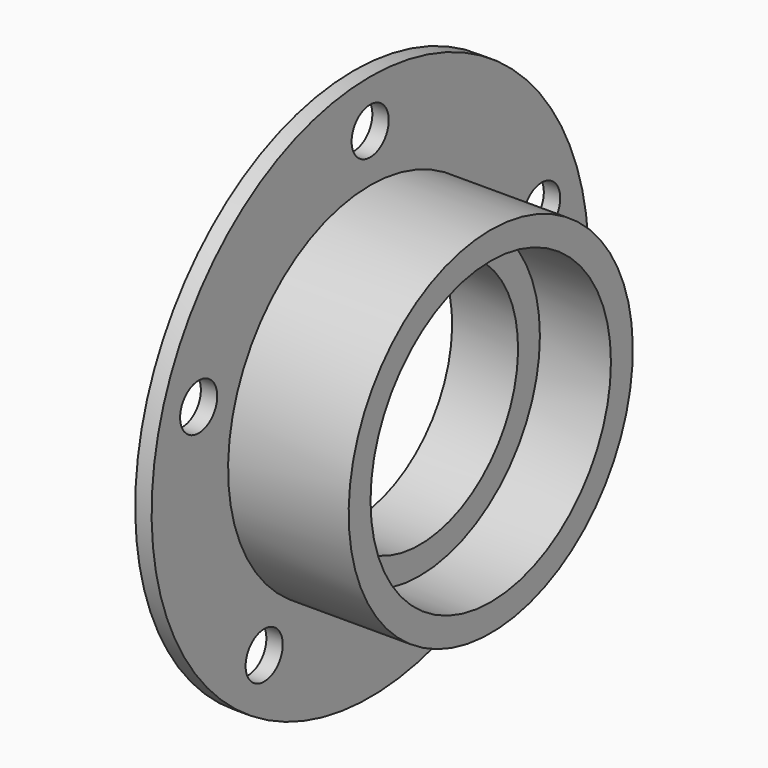
from build123d import *

# Parameters (mm, degrees)
F3_D     = 8.5
F3_DEPTH = 49.5
F3_TIP   = 2.5536576309


# Not quite as in the source:
# - a feature names something its author has since deleted; it is built from what else it names


with BuildPart() as f1:
    # F0 (on Front) → F1 (revolve)
    with BuildSketch(Plane.XZ):
        Polygon((-15.4332816247, 27.5), (-2.4332816247, 27.5), (-2.4332816247, 32.5), (-24.5, 32.5), (-24.5, 50), (-27.5, 50), (-27.5, 22.5), (-15.4332816247, 22.5), align=None)
    revolve(axis=Axis((-62.9697144032, 0, 0), (-1, 0, 0)))

    # F3
    with Locations(Plane(origin=(-27.5, 0, 0), x_dir=(0, -1, 0), z_dir=(-1, 0, 0))):
        with Locations((0, 41.25), (39.2310812972, 12.746951018), (24.2461416571, -33.371951018), (-24.2461416571, -33.371951018), (-39.2310812972, 12.746951018)):
            Hole(F3_D / 2, depth=F3_DEPTH)
            with Locations((0, 0, -(F3_DEPTH + F3_TIP / 2))):  # 118° drill point
                Cone(0, F3_D / 2, F3_TIP, mode=Mode.SUBTRACT)


solid = f1.part
